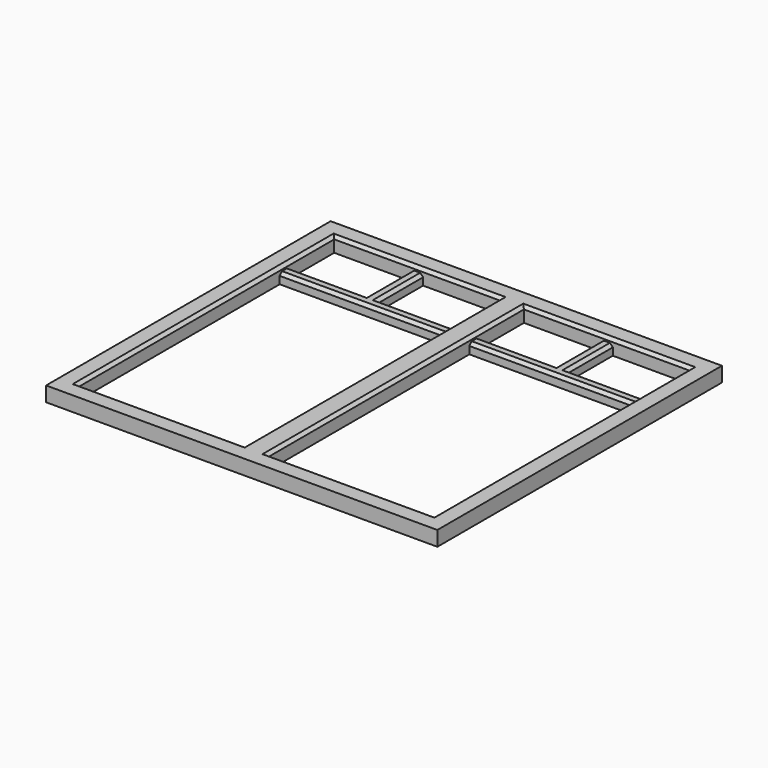
from build123d import *

# Parameters (mm, degrees)
F0_W      = 1320
F0_H      = 1200
F1_DEPTH  = 50
F2_DEPTH  = 35
F3_SIZE   = 10
F3_2_SIZE = 10
F3_3_SIZE = 10


with BuildPart() as f1:
    # F0 (on Top) → F1 (new body)
    with BuildSketch(Plane.XY):
        with Locations((220.3141621128, 45.2047318473)):
            Rectangle(F0_W, F0_H)
        Polygon((-379.6858378872, -494.7952681527), (-379.6858378872, 355.2047318473), (-379.6858378872, 395.2047318473), (-379.6858378872, 585.2047318473), (-119.6858378872, 585.2047318473), (-79.6858378872, 585.2047318473), (180.3141621128, 585.2047318473), (180.3141621128, 395.2047318473), (180.3141621128, 355.2047318473), (180.3141621128, -494.7952681527), align=None, mode=Mode.SUBTRACT)
        Polygon((260.3141621128, -494.7952681527), (260.3141621128, 355.2047318473), (260.3141621128, 395.2047318473), (260.3141621128, 585.2047318473), (520.3141621128, 585.2047318473), (560.3141621128, 585.2047318473), (820.3141621128, 585.2047318473), (820.3141621128, 395.2047318473), (820.3141621128, 355.2047318473), (820.3141621128, -494.7952681527), align=None, mode=Mode.SUBTRACT)
    extrude(amount=F1_DEPTH)

    # F3
    f3_edges = [f1.edges().sort_by_distance(p)[0] for p in [
        (-379.685838, 45.204732, 50),
        (-99.685838, 585.204732, 50),
        (180.314162, 45.204732, 50),
        (260.314162, 45.204732, 50),
        (540.314162, 585.204732, 50),
        (820.314162, 45.204732, 50),
        (540.314162, -494.795268, 50),
        (-99.685838, -494.795268, 50),
    ]]
    chamfer(f3_edges, length=F3_SIZE)


with BuildPart() as f2:
    # F0 (on Top) → F2 (new body)
    with BuildSketch(Plane.XY):
        Polygon((-379.6858378872, 395.2047318473), (-379.6858378872, 355.2047318473), (180.3141621128, 355.2047318473), (180.3141621128, 395.2047318473), (-79.6858378872, 395.2047318473), (-79.6858378872, 585.2047318473), (-119.6858378872, 585.2047318473), (-119.6858378872, 395.2047318473), align=None)
    extrude(amount=F2_DEPTH)

    # F3#2
    f3_2_edges = [f2.edges().sort_by_distance(p)[0] for p in [
        (-99.685838, 355.204732, 35),
        (50.314162, 395.204732, 35),
        (-79.685838, 490.204732, 35),
        (-119.685838, 490.204732, 35),
        (-249.685838, 395.204732, 35),
    ]]
    chamfer(f3_2_edges, length=F3_2_SIZE)


with BuildPart() as f2b:
    # F0 (on Top) → F2, piece 2 (new body)
    with BuildSketch(Plane.XY):
        Polygon((260.3141621128, 395.2047318473), (260.3141621128, 355.2047318473), (820.3141621128, 355.2047318473), (820.3141621128, 395.2047318473), (560.3141621128, 395.2047318473), (560.3141621128, 585.2047318473), (520.3141621128, 585.2047318473), (520.3141621128, 395.2047318473), align=None)
    extrude(amount=F2_DEPTH)

    # F3#3
    f3_3_edges = [f2b.edges().sort_by_distance(p)[0] for p in [
        (540.314162, 355.204732, 35),
        (390.314162, 395.204732, 35),
        (560.314162, 490.204732, 35),
        (690.314162, 395.204732, 35),
        (520.314162, 490.204732, 35),
    ]]
    chamfer(f3_3_edges, length=F3_3_SIZE)


solid = Compound([f1.part, f2.part, f2b.part])
